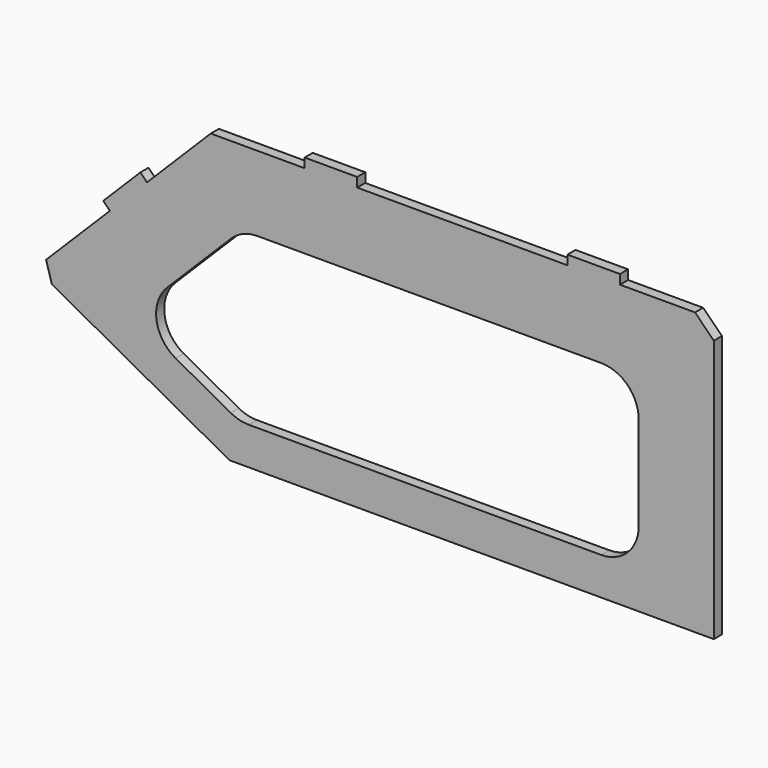
from build123d import *

# Parameters (mm, degrees)
F1_DEPTH = 3.429


# Not quite as in the source:
# - ends of sketch curves that miss each other by under 0.0002 mm in the source are joined


with BuildPart() as f1:
    # F0 (on Front) → F1 (new body)
    with BuildSketch(Plane.XZ):
        Polygon((-357.469059, -352.4197422), (-375.249059, -352.4197422), (-375.249059, -355.5947422), (-406.999059, -355.5947422), (-428.5679516, -377.1636348), (-430.8130322, -374.9185542), (-443.3853718, -387.4909192), (-441.1403166, -389.7359998), (-462.7092092, -411.3048924), (-460.7568382, -417.970716), (-400.649059, -450.8447422), (-236.819059, -450.8447422), (-236.819059, -361.9447422), (-243.169059, -355.5947422), (-268.569059, -355.5947422), (-268.569059, -352.4197422), (-286.349059, -352.4197422), (-286.349059, -355.5947422), (-357.469059, -355.5947422), align=None)
        with BuildLine():
            ThreePointArc((-418.8754328238, -426.4010670387), (-425.3527857587, -417.0618193312), (-421.7617140211, -406.2784129789))
            Line((-421.7617140211, -406.2784129789), (-400.1977772, -384.7144706))
            ThreePointArc((-400.1977772, -384.7144706), (-396.0776022944, -381.9614687005), (-391.217531, -380.9947422))
            Line((-391.217531, -380.9947422), (-274.919059, -380.9947422))
            ThreePointArc((-274.919059, -380.9947422), (-265.9388028789, -384.7144860789), (-262.219059, -393.6947422))
            Line((-262.219059, -393.6947422), (-262.219059, -425.4447422))
            ThreePointArc((-262.219059, -425.4447422), (-265.9388028789, -434.4249983211), (-274.919059, -438.1447422))
            Line((-274.919059, -438.1447422), (-394.1569714, -438.1447422))
            ThreePointArc((-394.1569714, -438.1447422), (-397.3019244332, -437.7491832852), (-400.250969717, -436.5871469904))
            Line((-400.250969717, -436.5871469904), (-418.8754328238, -426.4010670387))
        make_face(mode=Mode.SUBTRACT)
    extrude(amount=F1_DEPTH)


solid = f1.part
